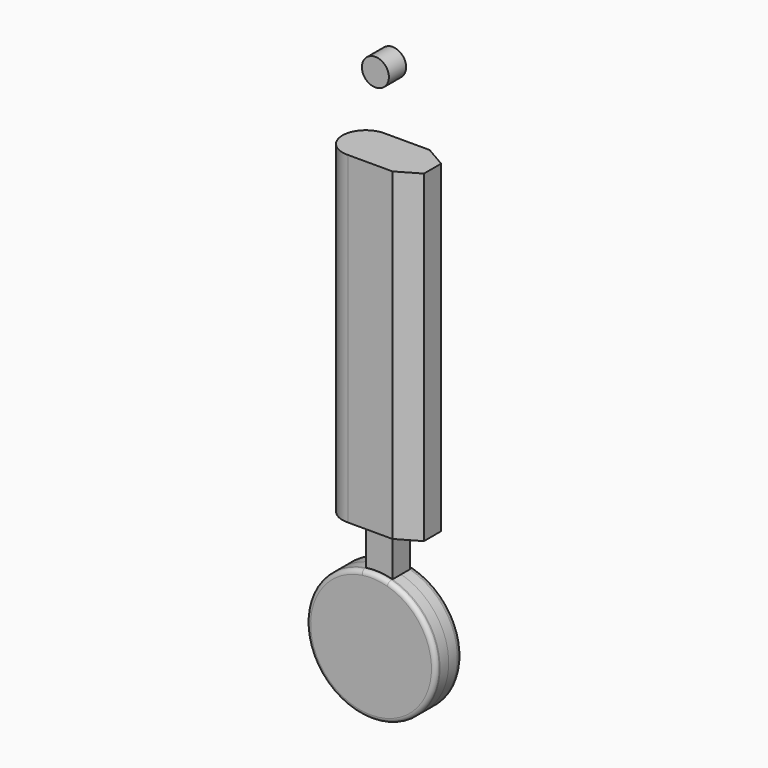
from build123d import *

# Parameters (mm, degrees)
F1_DEPTH = 12.7
F0_R     = 15.875
F2_DEPTH = 12.7
F3_DEPTH = 19.05
F5_DEPTH = 381
F6_R     = 5.08


with BuildPart() as f1:
    # F0 (on Front) → F1 (new body, symmetric)
    with BuildSketch(Plane.XZ):
        Polygon((57.15, 212.0332655495), (-19.05, 212.0332655495), (-19.05, -168.9667344505), (-11.0213747248, -168.9667344505), (0, -168.9667344505), (17.0811599865, -168.9667344505), (20.2070903033, -168.9667344505), (57.15, -168.9667344505), align=None)
        with BuildLine():
            Line((0, -168.9667344505), (-11.0213747248, -168.9667344505))
            Line((-11.0213747248, -168.9667344505), (-11.0213747248, -218.6437752822))
            ThreePointArc((-11.0213747248, -218.6437752822), (4.6928199973, -217.9871529405), (20.2070903033, -220.5706555117))
            Line((20.2070903033, -220.5706555117), (20.2070903033, -168.9667344505))
            Line((20.2070903033, -168.9667344505), (17.0811599865, -168.9667344505))
            Line((17.0811599865, -168.9667344505), (0, -168.9667344505))
        make_face()
    extrude(amount=F1_DEPTH, both=True)



with BuildPart() as f1b:
    # F0 (on Front) → F1, piece 2 (new body, symmetric)
    with BuildSketch(Plane.XZ):
        with BuildLine():
            Line((-11.0213747248, -232.3558569366), (-11.0213747248, -218.6437752822))
            ThreePointArc((-11.0213747248, -218.6437752822), (-49.8327765932, -351.6891443779), (76.2, -294.0425106773))
            ThreePointArc((76.2, -294.0425106773), (60.6061889625, -247.8545267481), (20.2070903033, -220.5706555117))
            Line((20.2070903033, -220.5706555117), (20.2070903033, -232.3558569366))
            Line((20.2070903033, -232.3558569366), (-11.0213747248, -232.3558569366))
        make_face()
    extrude(amount=F1_DEPTH, both=True)


with BuildPart() as f2:
    # F0 (on Front) → F2 (new body, symmetric)
    with BuildSketch(Plane.XZ):
        with Locations((0, 298.6241839262)):
            Circle(F0_R)
    extrude(amount=F2_DEPTH, both=True)


with BuildPart() as f1_1:
    add(f1.part)

    add(f1b.part)  # F3 merges F1b
    # F0 (on Front) → F3 (join, symmetric)
    with BuildSketch(Plane.XZ):
        with BuildLine():
            Line((-11.0213747248, -232.3558569366), (-11.0213747248, -218.6437752822))
            ThreePointArc((-11.0213747248, -218.6437752822), (-49.8327765932, -351.6891443779), (76.2, -294.0425106773))
            ThreePointArc((76.2, -294.0425106773), (60.6061889625, -247.8545267481), (20.2070903033, -220.5706555117))
            Line((20.2070903033, -220.5706555117), (20.2070903033, -232.3558569366))
            Line((20.2070903033, -232.3558569366), (-11.0213747248, -232.3558569366))
        make_face()
        with BuildLine():
            ThreePointArc((20.2070903033, -220.5706555117), (4.6928199973, -217.9871529405), (-11.0213747248, -218.6437752822))
            Line((-11.0213747248, -218.6437752822), (-11.0213747248, -232.3558569366))
            Line((-11.0213747248, -232.3558569366), (20.2070903033, -232.3558569366))
            Line((20.2070903033, -232.3558569366), (20.2070903033, -220.5706555117))
        make_face()
    extrude(amount=F3_DEPTH, both=True)

    # F4 (on face) → F5 (join, through all)
    with BuildSketch(Plane(origin=(0, 0, -168.9667344505), x_dir=(1, 0, 0), z_dir=(0, 0, -1))):
        with BuildLine():
            Line((31.8119843732, 27.3289101429), (-20.3755640355, 27.3289101429))
            ThreePointArc((-20.3755640355, 27.3289101429), (-48.8921323698, 0), (-20.3755640355, -27.3289101429))
            Line((-20.3755640355, -27.3289101429), (31.8119843732, -27.3289101429))
            Line((31.8119843732, -27.3289101429), (57.15, -12.7))
            Line((57.15, -12.7), (20.2070903033, -12.7))
            Line((20.2070903033, -12.7), (20.2070903033, 12.7))
            Line((20.2070903033, 12.7), (57.15, 12.7))
            Line((57.15, 12.7), (31.8119843732, 27.3289101429))
        make_face()
        Polygon((57.15, 0), (57.15, 12.7), (20.2070903033, 12.7), (20.2070903033, -12.7), (57.15, -12.7), align=None)
    extrude(amount=-F5_DEPTH)

    # F6
    f6_edges = [f1_1.edges().sort_by_distance(p)[0] for p in [
        (-76.2, -19.05, -294.042511),
        (-76.2, 19.05, -294.042511),
    ]]
    fillet(f6_edges, radius=F6_R)


solid = Compound([f2.part, f1_1.part])
